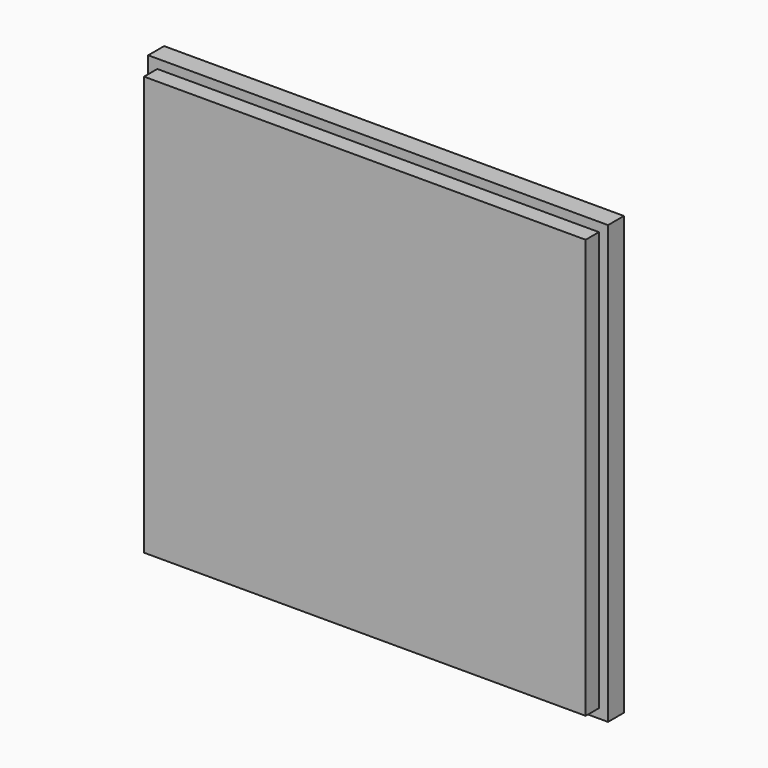
from build123d import *

# Parameters (mm, degrees)
F0_W     = 125.2775639296
F0_H     = 9.2387646437
F1_DEPTH = 2438.4
F2_DEPTH = 2438.4
F3_DEPTH = 101.6
F4_T     = -50.8
F5_DEPTH = 152.4


with BuildPart() as f1:
    # F0 (on Top) → F1 (new body)
    with BuildSketch(Plane.XY):
        with Locations((10.1626291871, 61.5301206708)):
            Rectangle(F0_W, F0_H)
    extrude(amount=F1_DEPTH)

    # F2 (add): a face of the model
    f2_faces = [f1.faces().sort_by_distance(p)[0] for p in [
        (-52.4761527777, 61.5301206708, 1219.2),
    ]]
    extrude(f2_faces, amount=F2_DEPTH)

    # F3 (add): a face of the model
    f3_faces = [f1.faces().sort_by_distance(p)[0] for p in [
        (-1209.0373708129, 66.1495029926, 1219.2),
    ]]
    extrude(f3_faces, amount=F3_DEPTH)

    # F4
    f4_openings = [f1.faces().sort_by_distance(p)[0] for p in [
        (-1209.037371, 56.910738, 1219.2),
    ]]
    offset(amount=F4_T, openings=f4_openings)

    # F5 (add): a face of the model
    f5_faces = [f1.faces().sort_by_distance(p)[0] for p in [
        (-1209.0373708129, 116.9495029926, 1219.2),
    ]]
    extrude(f5_faces, amount=F5_DEPTH)


solid = f1.part
